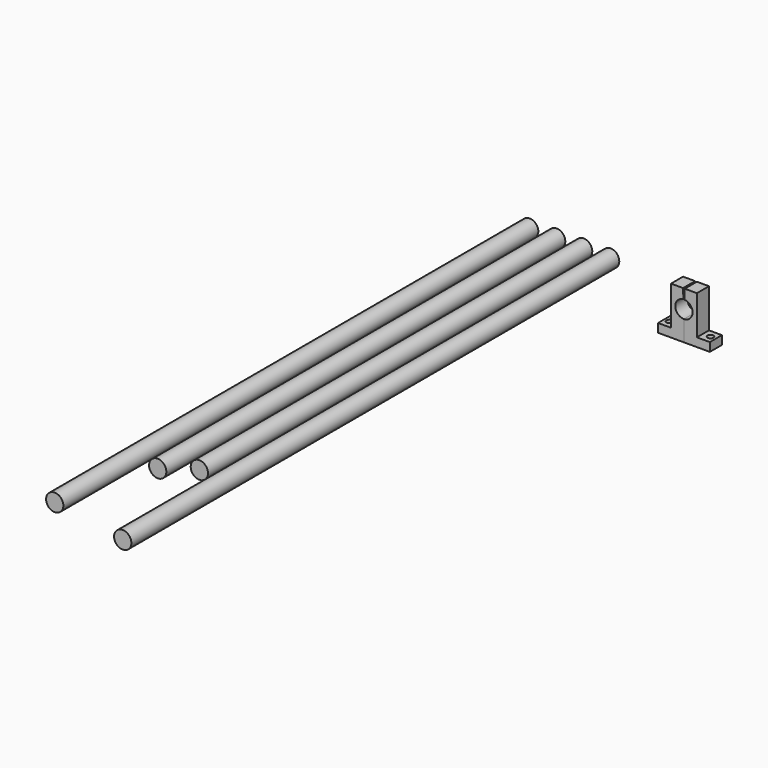
from build123d import *
from build123d import SkipClean  # not in build123d's __all__

# Parameters (mm, degrees)
F1_DEPTH  = 14
F2_R      = 2.75
F3_DEPTH  = 25
F5_DEPTH  = 25
F7_R      = 8
F8_DEPTH  = 550
F9_DEPTH  = 462
F10_DEPTH = 445
F11_DEPTH = 565


with BuildPart() as f1:
    # F0 (on Front) → F1 (new body)
    with BuildSketch(Plane.XZ):
        with BuildLine():
            Line((-24, 8), (-24, 0))
            Line((-24, 0), (0, 0))
            Line((0, 0), (0, 19))
            ThreePointArc((0, 19), (-8, 27), (0, 35))
            Line((0, 35), (0, 44))
            Line((0, 44), (-12, 44))
            Line((-12, 44), (-12, 8))
            Line((-12, 8), (-24, 8))
        make_face()
    extrude(amount=F1_DEPTH)

    # F2 (on face) → F3 (cut)
    with BuildSketch(Plane.XY.offset(8)):
        with Locations((-19, -7)):
            Circle(F2_R)
    extrude(amount=-F3_DEPTH, mode=Mode.SUBTRACT)

    # F4 (on face) → F5 (cut)
    with BuildSketch(Plane.XZ.offset(14)):
        with BuildLine():
            Line((0, 44), (-0.8, 44))
            Line((-0.8, 44), (-0.4997557997, 34.984375))
            ThreePointArc((-0.4997557997, 34.984375), (-0.25, 34.9960927959), (0, 35))
            Line((0, 35), (0, 44))
        make_face()
    extrude(amount=-F5_DEPTH, mode=Mode.SUBTRACT)

    # F6: F1 across face


with BuildPart() as f1_1:
    add(f1.part, clean=False)
    with SkipClean():  # cleaning this boolean's faces spoils the solid; the shape is the same uncleaned
        add(f1.part.mirror(Plane(origin=(0, -7, 9.5), x_dir=(0, 1, 0), z_dir=(1, 0, 0))), clean=False)


with BuildPart() as f8:
    # F7 (on Front) → F8 (new body)
    with BuildSketch(Plane.XZ):
        with Locations((-154.0818959475, 37.2658409178)):
            Circle(F7_R)
    extrude(amount=F8_DEPTH)


with BuildPart() as f9:
    # F7 (on Front) → F9 (new body)
    with BuildSketch(Plane.XZ):
        with Locations((-129.0818959475, 37.2658409178)):
            Circle(F7_R)
    extrude(amount=F9_DEPTH)


with BuildPart() as f10:
    # F7 (on Front) → F10 (new body)
    with BuildSketch(Plane.XZ):
        with Locations((-104.0818959475, 37.2658409178)):
            Circle(F7_R)
    extrude(amount=F10_DEPTH)


with BuildPart() as f11:
    # F7 (on Front) → F11 (new body)
    with BuildSketch(Plane.XZ):
        with Locations((-79.0818959475, 37.2658409178)):
            Circle(F7_R)
    extrude(amount=F11_DEPTH)


solid = Compound([f1_1.part, f8.part, f9.part, f10.part, f11.part])
